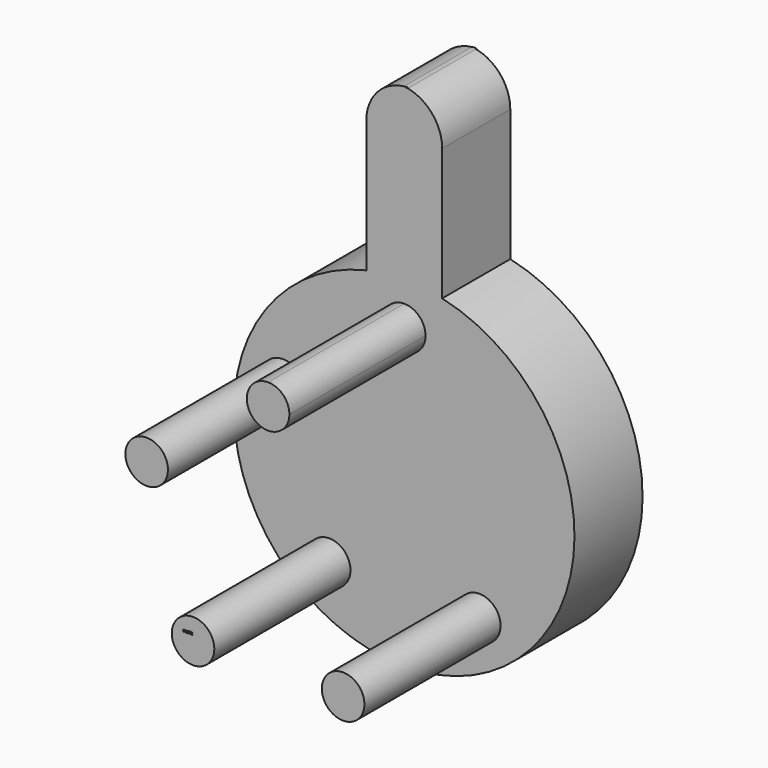
from build123d import *

# Parameters (mm, degrees)
F1_DEPTH     = 12.7
F2_R         = 3.175
F3_DEPTH     = 25.4
F4_TEXT_SIZE = 0.5982143597
F5_DEPTH     = 5.715


# Not quite as in the source:
# - a feature names something its author has since deleted; it is built from what else it names
# - Text() gives the source's letters only with a copy of the font that has no kerning and outlines rounded to 1/6400 em; it was checked with that copy


with BuildPart() as f1:
    # F0 (on Front) → F1 (new body)
    with BuildSketch(Plane.XZ):
        with BuildLine():
            ThreePointArc((-5.661085248, 24.7611008199), (-15.8330103692, -19.8614144171), (25.4, 0))
            ThreePointArc((25.4, 0), (19.8614144171, 15.8330103692), (5.661085248, 24.7611008199))
            ThreePointArc((5.661085248, 24.7611008199), (2.8485118197, 25.239769817), (0, 25.4))
            ThreePointArc((0, 25.4), (-2.8485118197, 25.239769817), (-5.661085248, 24.7611008199))
        make_face()
        with BuildLine():
            ThreePointArc((0, 25.4), (2.8485118197, 25.239769817), (5.661085248, 24.7611008199))
            Line((5.661085248, 24.7611008199), (5.661085248, 44.45))
            ThreePointArc((5.661085248, 44.45), (4.0385110102, 48.6895690421), (0, 50.7625190269))
            Line((0, 50.7625190269), (0, 25.4))
        make_face()
        with BuildLine():
            Line((-5.661085248, 44.45), (-5.661085248, 24.7611008199))
            ThreePointArc((-5.661085248, 24.7611008199), (-2.8485118197, 25.239769817), (0, 25.4))
            Line((0, 25.4), (0, 50.7625190269))
            ThreePointArc((0, 50.7625190269), (-4.0385110102, 48.6895690421), (-5.661085248, 44.45))
        make_face()
    extrude(amount=F1_DEPTH)

    # F2 (on face) → F3 (join)
    with BuildSketch(Plane.XZ.offset(12.7)):
        with BuildLine():
            ThreePointArc((0, 22.225), (-2.2450640303, 16.8049359697), (3.175, 19.05))
            ThreePointArc((3.175, 19.05), (2.2450640303, 21.2950640303), (0, 22.225))
        make_face()
        with Locations((-18.1176266354, 5.8867737428)):
            Circle(F2_R)
        with Locations((11.1973090562, -15.4117737428)):
            Circle(F2_R)
        with Locations((-11.1973090562, -15.4117737428)):
            Circle(F2_R)
    extrude(amount=F3_DEPTH)

    # F4 (on face) → F5 (cut)
    with BuildSketch(Plane.XZ.offset(38.1)):
        with Locations((-12.7662243322, -14.6501576528)):
            Text('penis', F4_TEXT_SIZE, font='Open Sans', text_align=(TextAlign.LEFT, TextAlign.BOTTOM))
    extrude(amount=-F5_DEPTH, mode=Mode.SUBTRACT)


with BuildPart() as f1b:
    # F0 (on Front) → F1, piece 2 (new body)
    with BuildSketch(Plane.XZ):
        with BuildLine():
            Line((0, 50.8), (0, 50.7625190269))
            ThreePointArc((0, 50.7625190269), (0.3439479569, 50.790622833), (0.688914752, 50.8))
            Line((0.688914752, 50.8), (0, 50.8))
        make_face()
    extrude(amount=F1_DEPTH)


solid = Compound([f1.part, f1b.part])
